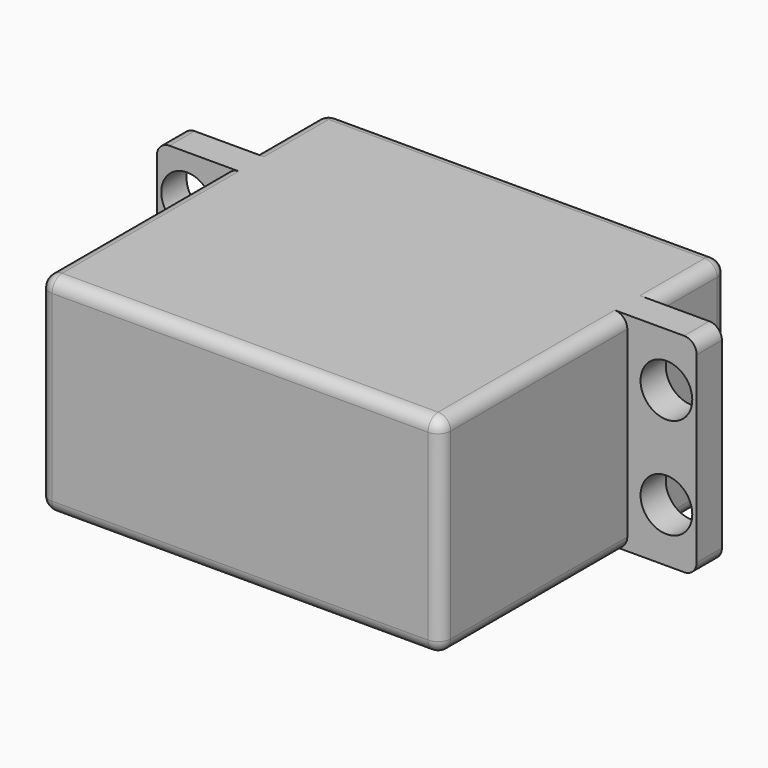
from build123d import *

# Parameters (mm, degrees)
F0_W      = 31.8
F0_H      = 7.4
F0_H_2    = 2.5
F0_H_3    = 18.5
F1_DEPTH  = 16.5
F4_R      = 2.05
F5_DEPTH  = 9.901
F6_R      = 5
F6_R_2    = 1.8453220601
F7_DEPTH  = 1.6
F8_SIZE   = 0.5
F9_R      = 1.8453220601
F10_DEPTH = 4
F12_DEPTH = 3.5
F13_R     = 1


# Not quite as in the source:
# - a feature names something its author has since deleted; it is built from what else it names


with BuildPart() as f1:
    # F0 (on Top) → F1 (new body)
    with BuildSketch(Plane.XY):
        with Locations((0, 10.5)):
            Rectangle(F0_W, F0_H)
        with Locations((0, 5.55)):
            Rectangle(F0_W, F0_H_2)
        with Locations((0, -4.95)):
            Rectangle(F0_W, F0_H_3)
        Polygon((-15.9, 4.3), (-15.9, 6.8), (-19, 6.8), (-21.4, 6.8), (-21.4, 4.3), (-19, 4.3), align=None)
        Polygon((19, 6.8), (15.9, 6.8), (15.9, 4.3), (19, 4.3), (21.4, 4.3), (21.4, 6.8), align=None)
    extrude(amount=F1_DEPTH)

    # F4 (on offset) → F5 (cut, through all)
    with BuildSketch(Plane.XZ.offset(-4.3)):
        with Locations((-19, 13.0433406178)):
            Circle(F4_R)
        with Locations((-19, 3.4566593822)):
            Circle(F4_R)
        with Locations((19, 12.25)):
            Circle(F4_R)
        with Locations((19, 4.25)):
            Circle(F4_R)
    extrude(amount=-F5_DEPTH, mode=Mode.SUBTRACT)

    # F6 (on face) → F7 (join)
    with BuildSketch(Plane(origin=(0, 14.2, 0), x_dir=(-1, 0, 0), z_dir=(0, 1, 0))):
        with Locations((-7.95, 8.25)):
            Circle(F6_R)
        with Locations((-7.95, 8.25)):
            Circle(F6_R_2, mode=Mode.SUBTRACT)
        with Locations((-7.95, 8.25)):
            Circle(F6_R_2)
    extrude(amount=F7_DEPTH)

    # F8
    f8_edges = [f1.edges().sort_by_distance(p)[0] for p in [
        (12.95, 15.8, 8.25),
    ]]
    chamfer(f8_edges, length=F8_SIZE)

    # F13
    f13_edges = [f1.edges().sort_by_distance(p)[0] for p in [
        (-15.9, -14.2, 8.25),
        (15.9, -14.2, 8.25),
        (0, -14.2, 0),
        (0, -14.2, 16.5),
        (0, 14.2, 16.5),
        (15.9, -4.95, 16.5),
        (15.9, -4.95, 0),
        (-15.9, -4.95, 0),
        (-15.9, -4.95, 16.5),
        (-15.9, 14.2, 8.25),
        (0, 14.2, 0),
        (15.9, 10.5, 0),
        (15.9, 10.5, 16.5),
        (21.4, 5.55, 16.5),
        (21.4, 5.55, 0),
        (-21.4, 5.55, 0),
        (-21.4, 5.55, 16.5),
        (-15.9, 10.5, 16.5),
        (-15.9, 10.5, 0),
        (15.9, 14.2, 8.25),
    ]]
    fillet(f13_edges, radius=F13_R)


with BuildPart() as f10:
    # F9 (on face) → F10 (new body)
    with BuildSketch(Plane(origin=(0, 15.8, 0), x_dir=(-1, 0, 0), z_dir=(0, 1, 0))):
        with Locations((-7.95, 8.25)):
            Circle(F9_R)
    extrude(amount=F10_DEPTH)

    # F11 (on face) → F12 (cut)
    with BuildSketch(Plane(origin=(0, 19.8, 0), x_dir=(-1, 0, 0), z_dir=(0, 1, 0))):
        with BuildLine():
            Line((-9.4809376593, 9.2802637472), (-8.8475196691, 9.2802637472))
            Line((-8.8475196691, 9.2802637472), (-8.760699031, 9.9077034073))
            ThreePointArc((-8.760699031, 9.9077034073), (-9.1621203443, 9.6413941844), (-9.4809376593, 9.2802637472))
        make_face()
        with BuildLine():
            Line((-9.7909627781, 8.376765748), (-9.2424067074, 8.6934747431))
            Line((-9.2424067074, 8.6934747431), (-9.4809376593, 9.2802637472))
            ThreePointArc((-9.4809376593, 9.2802637472), (-9.6954241028, 8.8489225382), (-9.7909627781, 8.376765748))
        make_face()
        with BuildLine():
            Line((-9.6077034073, 7.439300969), (-9.2909944122, 7.9878570397))
            Line((-9.2909944122, 7.9878570397), (-9.7909627781, 8.376765748))
            ThreePointArc((-9.7909627781, 8.376765748), (-9.7610428825, 7.8959700816), (-9.6077034073, 7.439300969))
        make_face()
        with BuildLine():
            Line((-8.9802637472, 6.7190623407), (-8.9802637472, 7.3524803309))
            Line((-8.9802637472, 7.3524803309), (-9.6077034073, 7.439300969))
            ThreePointArc((-9.6077034073, 7.439300969), (-9.3413941844, 7.0378796557), (-8.9802637472, 6.7190623407))
        make_face()
        with BuildLine():
            Line((-8.076765748, 6.4090372219), (-8.3934747431, 6.9575932926))
            Line((-8.3934747431, 6.9575932926), (-8.9802637472, 6.7190623407))
            ThreePointArc((-8.9802637472, 6.7190623407), (-8.5489225382, 6.5045758972), (-8.076765748, 6.4090372219))
        make_face()
        with BuildLine():
            Line((-7.139300969, 6.5922965927), (-7.6878570397, 6.9090055878))
            Line((-7.6878570397, 6.9090055878), (-8.076765748, 6.4090372219))
            ThreePointArc((-8.076765748, 6.4090372219), (-7.5959700816, 6.4389571175), (-7.139300969, 6.5922965927))
        make_face()
        with BuildLine():
            Line((-6.4190623407, 7.2197362528), (-7.0524803309, 7.2197362528))
            Line((-7.0524803309, 7.2197362528), (-7.139300969, 6.5922965927))
            ThreePointArc((-7.139300969, 6.5922965927), (-6.7378796557, 6.8586058156), (-6.4190623407, 7.2197362528))
        make_face()
        with BuildLine():
            Line((-6.1090372219, 8.123234252), (-6.6575932926, 7.8065252569))
            Line((-6.6575932926, 7.8065252569), (-6.4190623407, 7.2197362528))
            ThreePointArc((-6.4190623407, 7.2197362528), (-6.2045758972, 7.6510774618), (-6.1090372219, 8.123234252))
        make_face()
        with BuildLine():
            Line((-6.2922965927, 9.060699031), (-6.6090055878, 8.5121429603))
            Line((-6.6090055878, 8.5121429603), (-6.1090372219, 8.123234252))
            ThreePointArc((-6.1090372219, 8.123234252), (-6.1057680824, 8.1865796598), (-6.1046779399, 8.25))
            ThreePointArc((-6.1046779399, 8.25), (-6.1521943693, 8.6660629994), (-6.2922965927, 9.060699031))
        make_face()
        with BuildLine():
            Line((-6.9197362528, 9.7809376593), (-6.9197362528, 9.1475196691))
            Line((-6.9197362528, 9.1475196691), (-6.2922965927, 9.060699031))
            ThreePointArc((-6.2922965927, 9.060699031), (-6.5586058156, 9.4621203443), (-6.9197362528, 9.7809376593))
        make_face()
        with BuildLine():
            Line((-7.823234252, 10.0909627781), (-7.5065252569, 9.5424067074))
            Line((-7.5065252569, 9.5424067074), (-6.9197362528, 9.7809376593))
            ThreePointArc((-6.9197362528, 9.7809376593), (-7.3510774618, 9.9954241028), (-7.823234252, 10.0909627781))
        make_face()
        with BuildLine():
            Line((-8.760699031, 9.9077034073), (-8.2121429603, 9.5909944122))
            Line((-8.2121429603, 9.5909944122), (-7.823234252, 10.0909627781))
            ThreePointArc((-7.823234252, 10.0909627781), (-8.3040299184, 10.0610428825), (-8.760699031, 9.9077034073))
        make_face()
    extrude(amount=-F12_DEPTH, mode=Mode.SUBTRACT)


solid = Compound([f1.part, f10.part])
